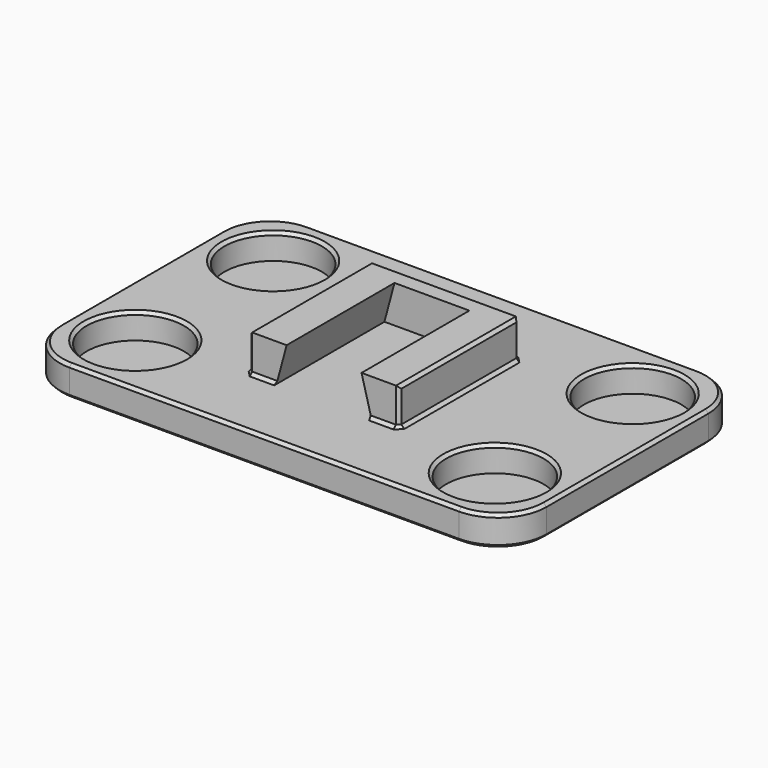
from build123d import *

# Parameters (mm, degrees)
F6_W      = 65
F6_H      = 40
F6_R      = 6.5
F7_DEPTH  = 4
F8_DEPTH  = 0.6
F6_W_2    = 20
F6_H_2    = 18
F6_H_3    = 2
F9_DEPTH  = 9
F11_DEPTH = 18
F12_R     = 6.5
F13_SIZE  = 0.4


with BuildPart() as f7:
    # F6 (on Top) → F7 (new body)
    with BuildSketch(Plane.XY):
        with Locations((32.5, 20)):
            Rectangle(F6_W, F6_H)
        with Locations((8.5, 8.5)):
            Circle(F6_R, mode=Mode.SUBTRACT)
        with Locations((56.5, 8.5)):
            Circle(F6_R, mode=Mode.SUBTRACT)
        with Locations((8.5, 31.5)):
            Circle(F6_R, mode=Mode.SUBTRACT)
        Polygon((22.5, 30), (42.5, 30), (42.5, 28), (42.5, 10), (22.5, 10), (22.5, 28), align=None, mode=Mode.SUBTRACT)
        with Locations((56.5, 31.5)):
            Circle(F6_R, mode=Mode.SUBTRACT)
    extrude(amount=F7_DEPTH)

    # F6 (on Top) → F8 (join)
    with BuildSketch(Plane.XY):
        with Locations((8.5, 31.5)):
            Circle(F6_R)
        with Locations((8.5, 8.5)):
            Circle(F6_R)
        with Locations((56.5, 8.5)):
            Circle(F6_R)
        with Locations((56.5, 31.5)):
            Circle(F6_R)
    extrude(amount=F8_DEPTH)

    # F6 (on Top) → F9 (join)
    with BuildSketch(Plane.XY):
        with Locations((32.5, 19)):
            Rectangle(F6_W_2, F6_H_2)
        with Locations((32.5, 29)):
            Rectangle(F6_W_2, F6_H_3)
    extrude(amount=F9_DEPTH)

    # F10 (on face) → F11 (cut)
    with BuildSketch(Plane.XZ.offset(-10)):
        Polygon((26.1602540378, 4), (38.8397459622, 4), (37.5, 9), (27.5, 9), align=None)
    extrude(amount=-F11_DEPTH, mode=Mode.SUBTRACT)

    # F12
    f12_edges = [f7.edges().sort_by_distance(p)[0] for p in [
        (0, 0, 2),
        (0, 40, 2),
        (65, 0, 2),
        (65, 40, 2),
    ]]
    fillet(f12_edges, radius=F12_R)

    # F13
    f13_edges = [f7.edges().sort_by_distance(p)[0] for p in [
        (0, 20, 0),
        (1.903806, 38.096194, 0),
        (1.903806, 1.903806, 0),
        (32.5, 40, 0),
        (32.5, 0, 0),
        (63.096194, 38.096194, 0),
        (63.096194, 1.903806, 0),
        (65, 20, 0),
        (22.5, 20, 4),
        (22.5, 10, 6.5),
        (22.5, 20, 9),
        (22.5, 30, 6.5),
        (42.5, 20, 4),
        (42.5, 30, 6.5),
        (42.5, 20, 9),
        (42.5, 10, 6.5),
        (50, 8.5, 4),
        (50, 31.5, 4),
        (2, 8.5, 4),
        (2, 31.5, 4),
        (32.5, 0, 4),
        (0, 20, 4),
        (1.903806, 38.096194, 4),
        (1.903806, 1.903806, 4),
        (32.5, 40, 4),
        (63.096194, 38.096194, 4),
        (63.096194, 1.903806, 4),
        (65, 20, 4),
        (32.5, 30, 4),
        (40.669873, 10, 4),
        (24.330127, 10, 4),
    ]]
    chamfer(f13_edges, length=F13_SIZE)


solid = f7.part
